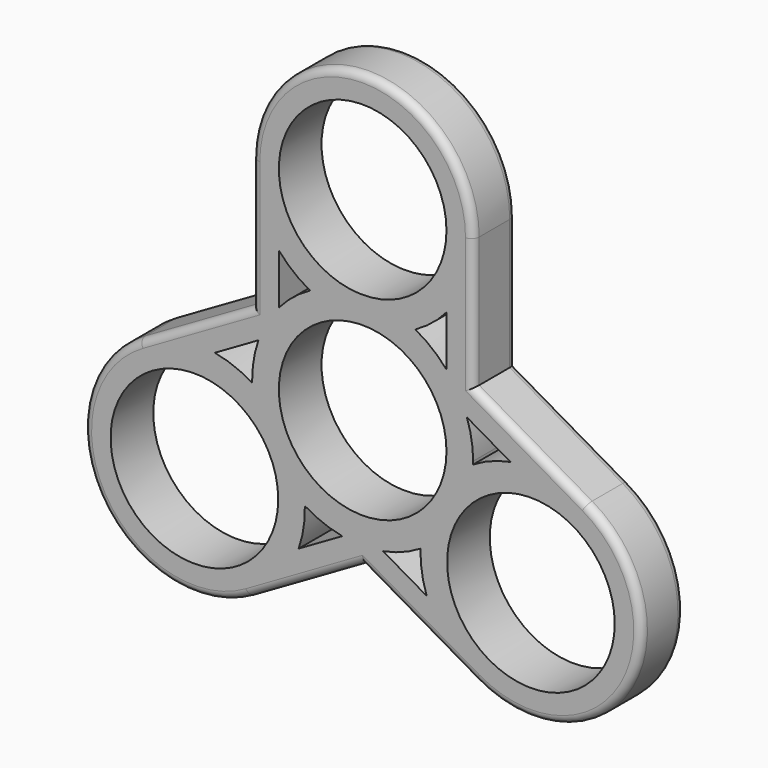
from build123d import *

# Parameters (mm, degrees)
F0_R     = 11
F1_DEPTH = 7
F2_R     = 1


# Not quite as in the source:
# - a feature names something its author has since deleted; it is built from what else it names


with BuildPart() as f1:
    # F0 (on Front) → F1 (new body)
    with BuildSketch(Plane.XZ):
        with BuildLine():
            ThreePointArc((14.5, 25.5), (0, 40), (-14.5, 25.5))
            Line((-14.5, 25.5), (-14.5, 8.3715789032))
            Line((-14.5, 8.3715789032), (-29.3336477965, -0.1926316451))
            ThreePointArc((-29.3336477965, -0.1926316451), (-34.6410161514, -20), (-14.8336477965, -25.3073683549))
            Line((-14.8336477965, -25.3073683549), (0, -16.7431578065))
            Line((0, -16.7431578065), (14.8336477965, -25.3073683549))
            ThreePointArc((14.8336477965, -25.3073683549), (34.6410161514, -20), (29.3336477965, -0.1926316451))
            Line((29.3336477965, -0.1926316451), (14.5, 8.3715789032))
            Line((14.5, 8.3715789032), (14.5, 25.5))
        make_face()
        with Locations((-22.0836477965, -12.75)):
            Circle(F0_R, mode=Mode.SUBTRACT)
        with BuildLine():
            ThreePointArc((-8.4021137105, -17.5526685347), (-7.7579062737, -14.9912339956), (-7.589017069, -12.355436857))
            ThreePointArc((-7.589017069, -12.355436857), (-5.2219051854, -13.5270730846), (-2.681534086, -14.2498903486))
            Line((-2.681534086, -14.2498903486), (-8.4021137105, -17.5526685347))
        make_face(mode=Mode.SUBTRACT)
        with BuildLine():
            ThreePointArc((-13.681534086, 4.8026685347), (-14.293919061, 2.4359552288), (-14.5, 0))
            ThreePointArc((-14.5, 0), (-14.4986576197, -0.1972998371), (-14.4946307275, -0.394563143))
            ThreePointArc((-14.4946307275, -0.394563143), (-16.8617426112, 0.7770730846), (-19.4021137105, 1.4998903486))
            Line((-19.4021137105, 1.4998903486), (-13.681534086, 4.8026685347))
        make_face(mode=Mode.SUBTRACT)
        with BuildLine():
            Line((8.4021137105, -17.5526685347), (2.681534086, -14.2498903486))
            ThreePointArc((2.681534086, -14.2498903486), (5.2219051854, -13.5270730846), (7.589017069, -12.355436857))
            ThreePointArc((7.589017069, -12.355436857), (7.7579062737, -14.9912339956), (8.4021137105, -17.5526685347))
        make_face(mode=Mode.SUBTRACT)
        with Locations((22.0836477965, -12.75)):
            Circle(F0_R, mode=Mode.SUBTRACT)
        Circle(F0_R, mode=Mode.SUBTRACT)
        with BuildLine():
            ThreePointArc((19.4021137105, 1.4998903486), (16.8617426112, 0.7770730846), (14.4946307275, -0.394563143))
            ThreePointArc((14.4946307275, -0.394563143), (14.4986576197, -0.1972998371), (14.5, 0))
            ThreePointArc((14.5, 0), (14.293919061, 2.4359552288), (13.681534086, 4.8026685347))
            Line((13.681534086, 4.8026685347), (19.4021137105, 1.4998903486))
        make_face(mode=Mode.SUBTRACT)
        with BuildLine():
            Line((-11, 9.4472218138), (-11, 16.0527781862))
            ThreePointArc((-11, 16.0527781862), (-9.1038363374, 14.214160911), (-6.9056136585, 12.75))
            ThreePointArc((-6.9056136585, 12.75), (-9.1038363374, 11.285839089), (-11, 9.4472218138))
        make_face(mode=Mode.SUBTRACT)
        with BuildLine():
            ThreePointArc((6.9056136585, 12.75), (9.1038363374, 14.214160911), (11, 16.0527781862))
            Line((11, 16.0527781862), (11, 9.4472218138))
            ThreePointArc((11, 9.4472218138), (9.1038363374, 11.285839089), (6.9056136585, 12.75))
        make_face(mode=Mode.SUBTRACT)
        with Locations((0, 25.5)):
            Circle(F0_R, mode=Mode.SUBTRACT)
    extrude(amount=F1_DEPTH)

    # F2
    f2_edges = [f1.edges().sort_by_distance(p)[0] for p in [
        (21.916824, -7, 4.089474),
        (14.5, -7, 16.935789),
        (14.5, 0, 16.935789),
        (21.916824, 0, 4.089474),
        (-7.416824, -7, -21.025263),
        (-21.916824, 0, 4.089474),
    ]]
    fillet(f2_edges, radius=F2_R)


solid = f1.part
